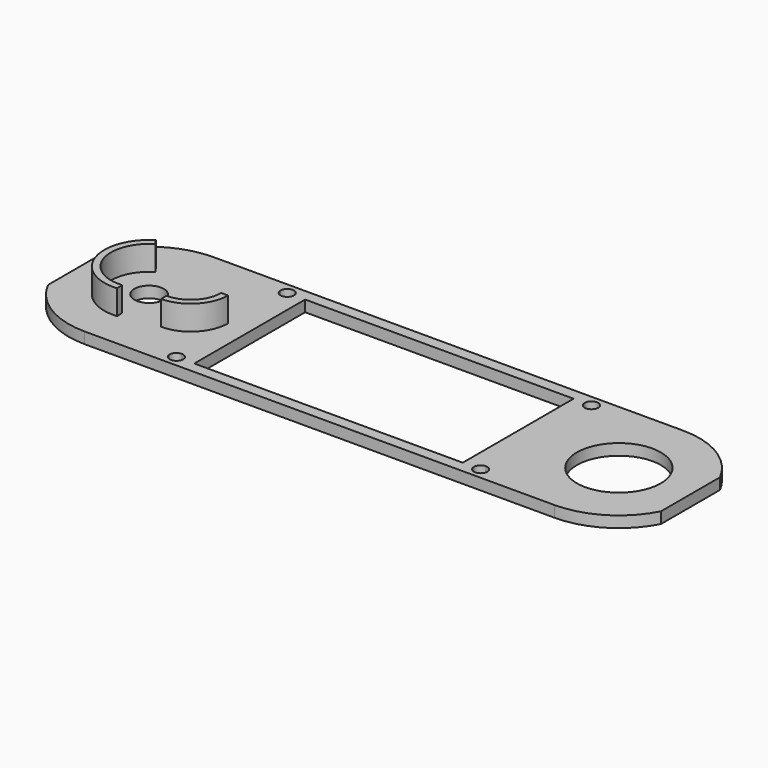
from build123d import *

# Parameters (mm, degrees)
F0_R     = 30
F0_R_2   = 10
F0_R_3   = 21.5
F0_R_4   = 18.75
F0_R_5   = 6.6
F1_DEPTH = 5
F3_DEPTH = 11


with BuildPart() as f1:
    # F0 (on Top) → F1 (new body)
    with BuildSketch(Plane.XY):
        with BuildLine():
            ThreePointArc((18.3030052177, -31), (31.2642622481, -17.8478543831), (36, 0))
            ThreePointArc((36, 0), (31.2978497092, 17.7888898917), (18.4197442455, 30.9307779069))
            ThreePointArc((18.4197442455, 30.9307779069), (9.5522770937, 34.7095664382), (0, 36))
            ThreePointArc((0, 36), (-18.7386337537, 30.7386337537), (-32, 16.4924225025))
            Line((-32, 16.4924225025), (-32, -16.4924225025))
            ThreePointArc((-32, -16.4924225025), (-18.7386337537, -30.7386337537), (0, -36))
            ThreePointArc((0, -36), (9.4868329805, -34.7275107084), (18.3030052177, -31))
        make_face()
        Circle(F0_R, mode=Mode.SUBTRACT)
        with BuildLine():
            ThreePointArc((242, 16.4924225025), (228.7386337537, 30.7386337537), (210, 36))
            ThreePointArc((210, 36), (200.4477229063, 34.7095664382), (191.5802557545, 30.9307779069))
            ThreePointArc((191.5802557545, 30.9307779069), (174.0000639573, -0.0678595955), (191.6969947823, -31))
            ThreePointArc((191.6969947823, -31), (200.5131670195, -34.7275107084), (210, -36))
            ThreePointArc((210, -36), (228.7386337537, -30.7386337537), (242, -16.4924225025))
            Line((242, -16.4924225025), (242, 16.4924225025))
        make_face()
        with Locations((210, 0)):
            Circle(F0_R, mode=Mode.SUBTRACT)
        Circle(F0_R)
        Circle(F0_R_2, mode=Mode.SUBTRACT)
        with Locations((210, 0)):
            Circle(F0_R)
        with Locations((210, 0)):
            Circle(F0_R_3, mode=Mode.SUBTRACT)
        with Locations((210, 0)):
            Circle(F0_R_3)
        with Locations((210, 0)):
            Circle(F0_R_4, mode=Mode.SUBTRACT)
        with BuildLine():
            ThreePointArc((19.6214168703, 36), (23.4046464655, 33.6633706545), (26.9125802938, 30.9307779069))
            Line((26.9125802938, 30.9307779069), (34, 30.9307779069))
            ThreePointArc((34, 30.9307779069), (37, 33.9307779069), (40, 30.9307779069))
            Line((40, 30.9307779069), (45, 30.9307779069))
            Line((45, 30.9307779069), (165, 30.9307779069))
            Line((165, 30.9307779069), (170, 30.9307779069))
            ThreePointArc((170, 30.9307779069), (173, 33.9307779069), (176, 30.9307779069))
            Line((176, 30.9307779069), (183.0874197062, 30.9307779069))
            ThreePointArc((183.0874197062, 30.9307779069), (186.5953535345, 33.6633706545), (190.3785831296, 36))
            Line((190.3785831296, 36), (19.6214168703, 36))
        make_face()
        with BuildLine():
            Line((34, -31), (26.83281573, -31))
            ThreePointArc((26.83281573, -31), (23.361269906, -33.693487032), (19.6214168703, -36))
            Line((19.6214168703, -36), (190.3785831296, -36))
            ThreePointArc((190.3785831296, -36), (186.638730094, -33.693487032), (183.16718427, -31))
            Line((183.16718427, -31), (176, -31))
            ThreePointArc((176, -31), (173, -34), (170, -31))
            Line((170, -31), (165, -31))
            Line((165, -31), (45, -31))
            Line((45, -31), (40, -31))
            ThreePointArc((40, -31), (37, -34), (34, -31))
        make_face()
        with BuildLine():
            Line((37, 27.9307779069), (37, 17.6635217327))
            ThreePointArc((37, 17.6635217327), (39.9874980463, 9.0553851381), (41, 0))
            ThreePointArc((41, 0), (39.9874980463, -9.0553851381), (37, -17.6635217327))
            Line((37, -17.6635217327), (37, -28))
            ThreePointArc((37, -28), (39.1213203436, -28.8786796564), (40, -31))
            Line((40, -31), (45, -31))
            Line((45, -31), (45, 30.9307779069))
            Line((45, 30.9307779069), (40, 30.9307779069))
            ThreePointArc((40, 30.9307779069), (39.1213203436, 28.8094575634), (37, 27.9307779069))
        make_face()
        with BuildLine():
            ThreePointArc((173, -17.6635217327), (169, 0), (173, 17.6635217327))
            Line((173, 17.6635217327), (173, 27.9307779069))
            ThreePointArc((173, 27.9307779069), (170.8786796564, 28.8094575634), (170, 30.9307779069))
            Line((170, 30.9307779069), (165, 30.9307779069))
            Line((165, 30.9307779069), (165, -31))
            Line((165, -31), (170, -31))
            ThreePointArc((170, -31), (170.8786796564, -28.8786796564), (173, -28))
            Line((173, -28), (173, -17.6635217327))
        make_face()
        Circle(F0_R_2)
        Circle(F0_R_5, mode=Mode.SUBTRACT)
        with BuildLine():
            ThreePointArc((18.4197442455, 30.9307779069), (31.2978497092, 17.7888898917), (36, 0))
            ThreePointArc((36, 0), (31.2642622481, -17.8478543831), (18.3030052177, -31))
            Line((18.3030052177, -31), (26.83281573, -31))
            ThreePointArc((26.83281573, -31), (32.6055594055, -24.8571417474), (37, -17.6635217327))
            Line((37, -17.6635217327), (37, 17.6635217327))
            ThreePointArc((37, 17.6635217327), (32.6375474194, 24.815126404), (26.9125802938, 30.9307779069))
            Line((26.9125802938, 30.9307779069), (18.4197442455, 30.9307779069))
        make_face()
        with BuildLine():
            Line((191.5802557545, 30.9307779069), (183.0874197062, 30.9307779069))
            ThreePointArc((183.0874197062, 30.9307779069), (177.3624525806, 24.815126404), (173, 17.6635217327))
            Line((173, 17.6635217327), (173, -17.6635217327))
            ThreePointArc((173, -17.6635217327), (177.3944405945, -24.8571417474), (183.16718427, -31))
            Line((183.16718427, -31), (191.6969947823, -31))
            ThreePointArc((191.6969947823, -31), (174.0000639573, -0.0678595955), (191.5802557545, 30.9307779069))
        make_face()
        with BuildLine():
            ThreePointArc((41, 0), (39.9874980463, 9.0553851381), (37, 17.6635217327))
            Line((37, 17.6635217327), (37, -17.6635217327))
            ThreePointArc((37, -17.6635217327), (39.9874980463, -9.0553851381), (41, 0))
        make_face()
        with BuildLine():
            Line((173, -17.6635217327), (173, 17.6635217327))
            ThreePointArc((173, 17.6635217327), (169, 0), (173, -17.6635217327))
        make_face()
        with BuildLine():
            ThreePointArc((0, 36), (9.5522770937, 34.7095664382), (18.4197442455, 30.9307779069))
            Line((18.4197442455, 30.9307779069), (26.9125802938, 30.9307779069))
            ThreePointArc((26.9125802938, 30.9307779069), (23.4046464655, 33.6633706545), (19.6214168703, 36))
            Line((19.6214168703, 36), (0, 36))
        make_face()
        with BuildLine():
            Line((210, 36), (190.3785831296, 36))
            ThreePointArc((190.3785831296, 36), (186.5953535345, 33.6633706545), (183.0874197062, 30.9307779069))
            Line((183.0874197062, 30.9307779069), (191.5802557545, 30.9307779069))
            ThreePointArc((191.5802557545, 30.9307779069), (200.4477229063, 34.7095664382), (210, 36))
        make_face()
        with BuildLine():
            Line((26.83281573, -31), (18.3030052177, -31))
            ThreePointArc((18.3030052177, -31), (9.4868329805, -34.7275107084), (0, -36))
            Line((0, -36), (19.6214168703, -36))
            ThreePointArc((19.6214168703, -36), (23.361269906, -33.693487032), (26.83281573, -31))
        make_face()
        with BuildLine():
            ThreePointArc((183.16718427, -31), (186.638730094, -33.693487032), (190.3785831296, -36))
            Line((190.3785831296, -36), (210, -36))
            ThreePointArc((210, -36), (200.5131670195, -34.7275107084), (191.6969947823, -31))
            Line((191.6969947823, -31), (183.16718427, -31))
        make_face()
        with BuildLine():
            ThreePointArc((37, -17.6635217327), (32.6055594055, -24.8571417474), (26.83281573, -31))
            Line((26.83281573, -31), (34, -31))
            ThreePointArc((34, -31), (34.8786796564, -28.8786796564), (37, -28))
            Line((37, -28), (37, -17.6635217327))
        make_face()
        with BuildLine():
            Line((176, -31), (183.16718427, -31))
            ThreePointArc((183.16718427, -31), (177.3944405945, -24.8571417474), (173, -17.6635217327))
            Line((173, -17.6635217327), (173, -28))
            ThreePointArc((173, -28), (175.1213203436, -28.8786796564), (176, -31))
        make_face()
        with BuildLine():
            Line((34, 30.9307779069), (26.9125802938, 30.9307779069))
            ThreePointArc((26.9125802938, 30.9307779069), (32.6375474194, 24.815126404), (37, 17.6635217327))
            Line((37, 17.6635217327), (37, 27.9307779069))
            ThreePointArc((37, 27.9307779069), (34.8786796564, 28.8094575634), (34, 30.9307779069))
        make_face()
        with BuildLine():
            ThreePointArc((173, 17.6635217327), (177.3624525806, 24.815126404), (183.0874197062, 30.9307779069))
            Line((183.0874197062, 30.9307779069), (176, 30.9307779069))
            ThreePointArc((176, 30.9307779069), (175.1213203436, 28.8094575634), (173, 27.9307779069))
            Line((173, 27.9307779069), (173, 17.6635217327))
        make_face()
    extrude(amount=F1_DEPTH)

    # F2 (on face) → F3 (join)
    with BuildSketch(Plane.XY.offset(5)):
        with BuildLine():
            ThreePointArc((32.2300370842, 0), (28.249548951, -9.6195118668), (18.6300370842, -13.6))
            Line((18.6300370842, -13.6), (18.6278837067, -16.5999992272))
            ThreePointArc((18.6278837067, -16.5999992272), (30.3708692945, -11.7408322103), (35.2300363114, 0.0021533775))
            Line((35.2300363114, 0.0021533775), (32.2300370842, 0))
        make_face()
        with BuildLine():
            ThreePointArc((1.4010723087, -16.9409777332), (-16.154736314, -5.264086135), (-8.8464426541, 14.5133013966))
            Line((-8.8464426541, 14.5133013966), (-10.5643945811, 16.9784386755))
            ThreePointArc((-10.5643945811, 16.9784386755), (-18.9787357989, -6.2800054738), (1.6467177805, -19.9309038698))
            Line((1.6467177805, -19.9309038698), (1.4010723087, -16.9409777332))
        make_face()
    extrude(amount=F3_DEPTH)


solid = f1.part
